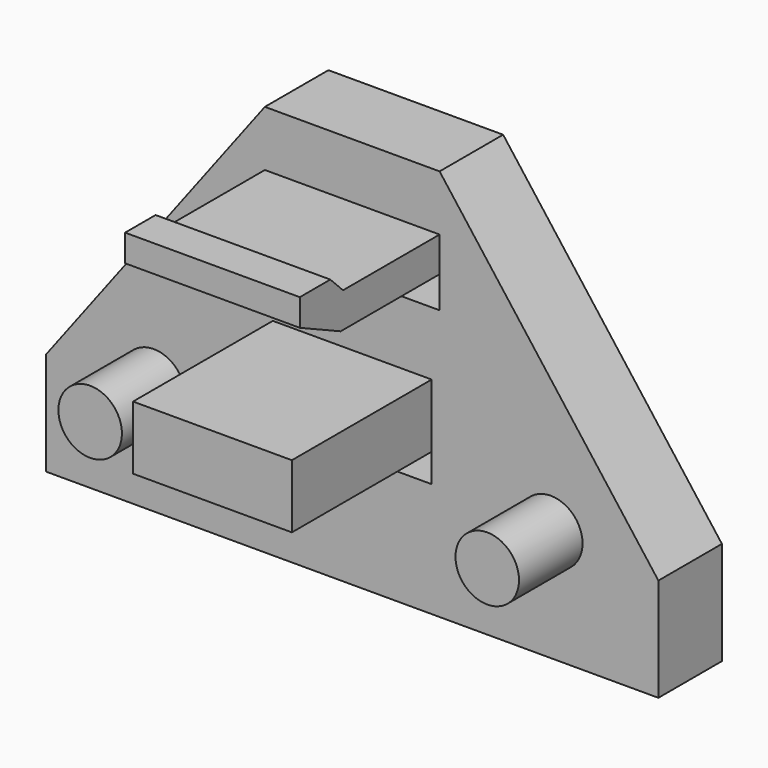
from build123d import *

# Parameters (mm, degrees)
F0_R         = 2
F1_DEPTH     = 5
F2_DEPTH     = 10
F0_W         = 5
F0_H         = 4
F0_W_2       = 5.5
F0_H_2       = 2.2
F3_DEPTH     = 16
F4_W         = 11
F4_H         = 3.4
F5_DEPTH     = 1
F6_SIZE      = 0.99999
F7_SIZE2     = 3.2167603808
F7_SIZE      = 1.5
F8_TEXT_SIZE = 7.2312248397
F9_DEPTH     = 0.5


# Not quite as in the source:
# - a fillet or chamfer is up to 0.001 mm smaller than in the source, because OpenCascade refuses the exact size
# - Text() gives the source's letters only with a copy of the font that has no kerning and outlines rounded to 1/6400 em; it was checked with that copy


with BuildPart() as f1:
    # F0 (on Front) → F1 (new body)
    with BuildSketch(Plane.XZ):
        Polygon((-5, -1.8), (-5, 0), (-5, 4), (0, 4), (0, 8), (-5.5, 8), (-5.5, 10), (-5.5, 12.2), (0, 12.2), (0, 15.7), (-5.5, 15.7), (-19.2751847208, -2.5), (-19.2751847208, -9), (0, -9), (0, -1.8), align=None)
        with Locations((-12.5, -2)):
            Circle(F0_R, mode=Mode.SUBTRACT)
        Polygon((5, 4), (5, 0), (5, -1.8), (0, -1.8), (0, -9), (19.2751847208, -9), (19.2751847208, -2.5), (5.5, 15.7), (0, 15.7), (0, 12.2), (5.5, 12.2), (5.5, 10), (5.5, 8), (0, 8), (0, 4), align=None)
        with Locations((12.5, -2)):
            Circle(F0_R, mode=Mode.SUBTRACT)
    extrude(amount=F1_DEPTH)

    # F0 (on Front) → F2 (join)
    with BuildSketch(Plane.XZ):
        with Locations((-12.5, -2)):
            Circle(F0_R)
        with Locations((12.5, -2)):
            Circle(F0_R)
    extrude(amount=F2_DEPTH)

    # F0 (on Front) → F3 (join)
    with BuildSketch(Plane.XZ):
        with Locations((2.5, 2)):
            Rectangle(F0_W, F0_H)
        with Locations((-2.5, 2)):
            Rectangle(F0_W, F0_H)
        with Locations((-2.75, 11.1)):
            Rectangle(F0_W_2, F0_H_2)
        with Locations((2.75, 11.1)):
            Rectangle(F0_W_2, F0_H_2)
    extrude(amount=F3_DEPTH)

    # F4 (on face) → F5 (join)
    with BuildSketch(Plane.XY.offset(12.2)):
        with Locations((0, -14.3)):
            Rectangle(F4_W, F4_H)
    extrude(amount=F5_DEPTH)

    # F6 (size 1 in the source; OpenCascade refuses exactly that, so slightly less here)
    f6_edges = [f1.edges().sort_by_distance(p)[0] for p in [
        (0, -12.6, 13.2),
    ]]
    chamfer(f6_edges, length=F6_SIZE)

    # F7
    f7_edges = [f1.edges().sort_by_distance(p)[0] for p in [
        (0, -16, 10),
    ]]
    f7_side = f1.faces().sort_by_distance((0, -16, 11.6))[0]
    chamfer(f7_edges, length=F7_SIZE, length2=F7_SIZE2, reference=f7_side)

    # F8 (on face) → F9 (cut)
    with BuildSketch(Plane(origin=(0, 0, 0), x_dir=(-1, 0, 0), z_dir=(0, 1, 0))):
        with Locations((-12.2377181623, 1.5915343642)):
            Text('SHANE', F8_TEXT_SIZE, font='Open Sans', font_style=FontStyle.BOLD, text_align=(TextAlign.LEFT, TextAlign.BOTTOM))
    extrude(amount=-F9_DEPTH, mode=Mode.SUBTRACT)


solid = f1.part
